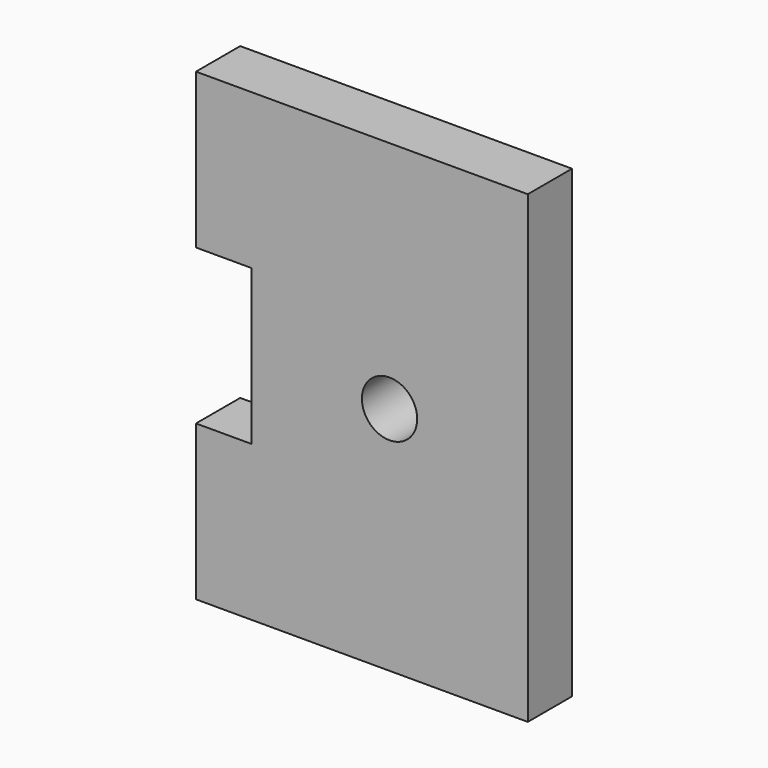
from build123d import *

# Parameters (mm, degrees)
F0_W     = 3.175
F0_H     = 8.89
F1_DEPTH = 3.175
F2_R     = 1.5875
F3_DEPTH = 3.176


# Not quite as in the source:
# - a feature names something its author has since deleted; it is built from what else it names


with BuildPart() as f1:
    # F0 (on Front) → F1 (new body)
    with BuildSketch(Plane.XZ):
        Polygon((9.525, 11.43), (9.525, 38.1), (-6.35, 38.1), (-6.35, 29.21), (-6.35, 20.32), (-6.35, 11.43), align=None)
        with Locations((-7.9375, 33.655)):
            Rectangle(F0_W, F0_H)
        with Locations((-7.9375, 15.875)):
            Rectangle(F0_W, F0_H)
    extrude(amount=F1_DEPTH)

    # F2 (on face) → F3 (cut, through all)
    with BuildSketch(Plane.XZ.offset(3.175)):
        with Locations((1.5875, 24.6701687584)):
            Circle(F2_R)
    extrude(amount=-F3_DEPTH, mode=Mode.SUBTRACT)


solid = f1.part
